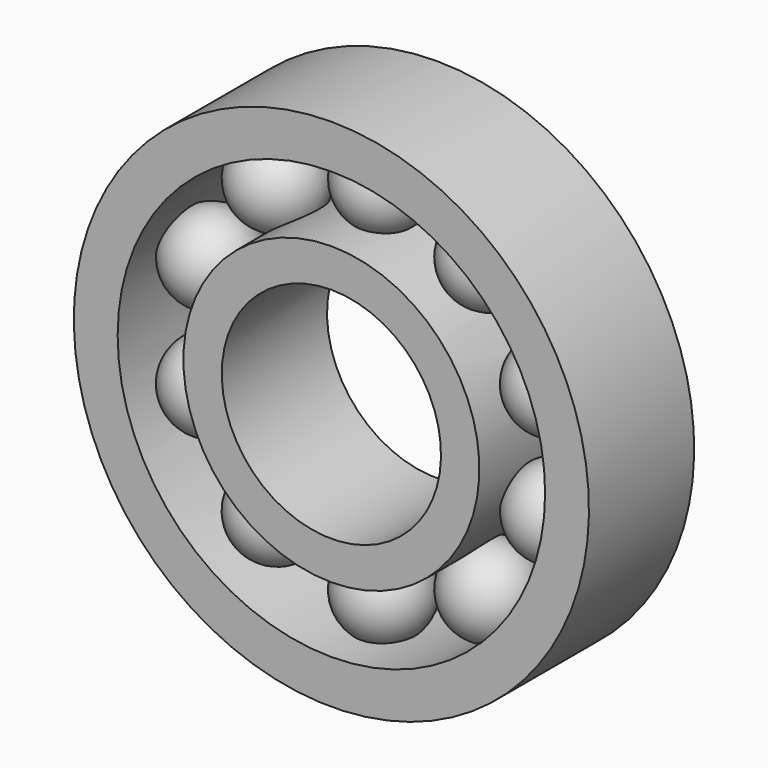
from build123d import *

# Parameters (mm, degrees)
F0_W     = 12
F0_H     = 4
F0_H_2   = 3.5
F6_COUNT = 10


with BuildPart() as f1:
    # F0 (on Right) → F1 (revolve)
    with BuildSketch(Plane.YZ):
        with Locations((-6, 21.5)):
            Rectangle(F0_W, F0_H)
    revolve(axis=Axis((0, -1.87192671, 0), (0, 1, 0)))



with BuildPart() as f1b:
    # F0 (on Right) → F1, piece 2 (revolve)
    with BuildSketch(Plane.YZ):
        with Locations((-6, 11.75)):
            Rectangle(F0_W, F0_H_2)
    revolve(axis=Axis((0, -1.87192671, 0), (0, 1, 0)))


with BuildPart() as f1_1:
    add(f1.part)

    add(f1b.part)  # F4 merges F1b
    # F3 (on offset) → F4 (revolve)
    with BuildSketch(Plane.XZ.offset(6)):
        with BuildLine():
            Line((0, 20.5), (0, 12.5))
            ThreePointArc((0, 12.5), (4, 16.5), (0, 20.5))
        make_face()
    revolve(axis=Axis((0, -6, 16.5), (0, 0, 1)))

    # F6: F1 ×10 about axis
    f6_axis = Axis((0, -7.2940571699, 0), (0, 1, 0))


with BuildPart() as f1_2:
    add(f1_1.part)
    for i in range(1, F6_COUNT):
        add(f1_1.part.rotate(f6_axis, i * 360 / F6_COUNT))


solid = f1_2.part
